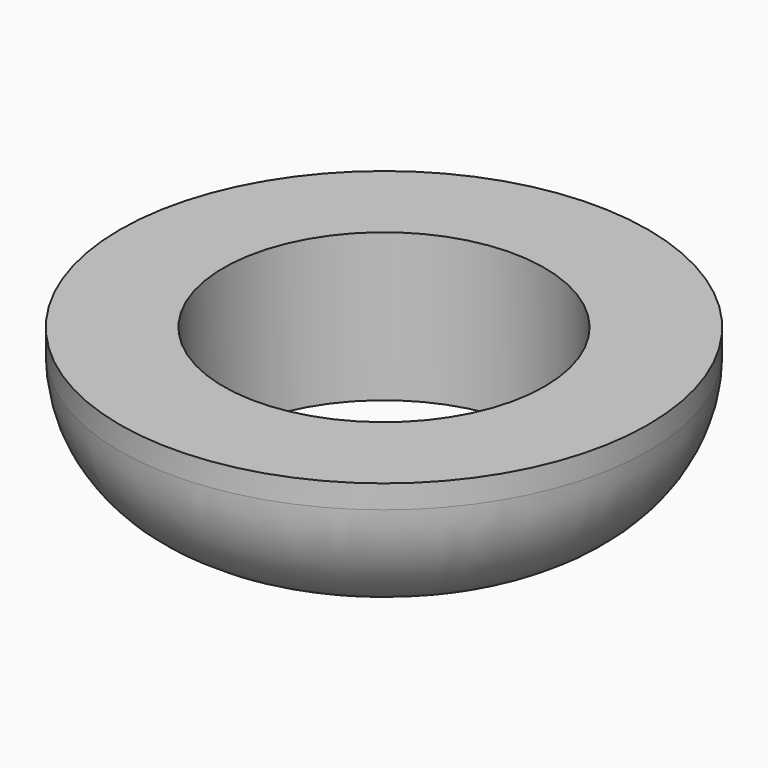
from build123d import *

# Parameters (mm, degrees)
F0_R     = 12.5
F0_R_2   = 7.6
F1_DEPTH = 7


# Not quite as in the source:
# - a fillet or chamfer that OpenCascade refuses, or shapes differently, is made with other operations: its cross-section is extruded or revolved along the edge and cut away or added


with BuildPart() as f1:
    # F0 (on Top) → F1 (new body)
    with BuildSketch(Plane.XY):
        Circle(F0_R)
        Circle(F0_R_2, mode=Mode.SUBTRACT)
    extrude(amount=-F1_DEPTH)

    # F2: fillet of radius 6 on 1 edges, made by hand

    # F2_s1 → F2_t2 (revolve, cut)
    with BuildSketch(Plane.XZ):
        with BuildLine():
            ThreePointArc((12.5, -1.1016951588), (11.1151923037, -4.9357530613), (7.6, -7))
            Line((7.6, -7), (12.5, -7))
            Line((12.5, -7), (12.5, -1.1016951588))
        make_face()
    revolve(axis=Axis((0, 0, -7), (0, 0, 1)), mode=Mode.SUBTRACT)


solid = f1.part
